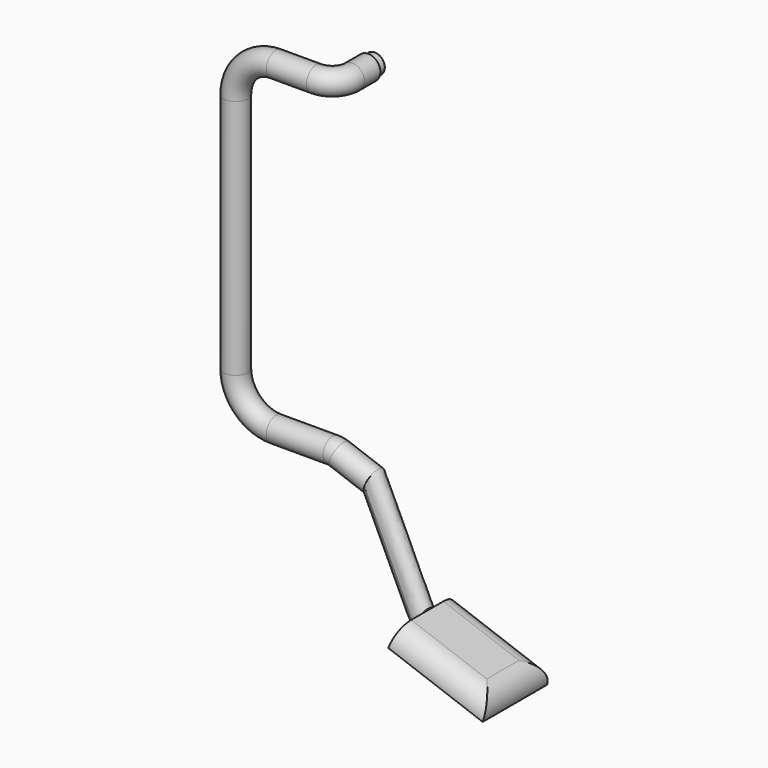
from build123d import *

# Parameters (mm, degrees)
F0_R      = 2.5
F1_DEPTH  = 2
F2_R      = 3
F5_R      = 3
F10_DEPTH = 1
F13_W     = 20
F13_H     = 5
F14_DEPTH = 25
F15_R     = 4.99999


# Not quite as in the source:
# - a fillet or chamfer is up to 0.001 mm smaller than in the source, because OpenCascade refuses the exact size


with BuildPart() as f1:
    # F0 (on Front) → F1 (new body)
    with BuildSketch(Plane.XZ):
        Circle(F0_R)
    extrude(amount=F1_DEPTH)

    # F4: sweep along a path in F3
    with BuildLine(Plane.XY) as f4_path:
        Line((0, -2), (0, -7))
        ThreePointArc((0, -7), (-1.4644660941, -10.5355339059), (-5, -12))
        Line((-5, -12), (-10, -12))
    # F2 (on face) → F4 (sweep)
    with BuildSketch(Plane.XZ.offset(2)):
        Circle(F2_R)
    sweep(path=f4_path.line)

    # F8: sweep along a path in F7
    with BuildLine(Plane.XZ.offset(12)) as f8_path:
        Line((-10, 0), (-15, 0))
        ThreePointArc((-15, 0), (-22.0710678119, -2.9289321881), (-25, -10))
        Line((-25, -10), (-25, -70))
        ThreePointArc((-25, -70), (-22.0710678119, -77.0710678119), (-15, -80))
        Line((-15, -80), (-0.8816349035, -80))
        ThreePointArc((-0.8816349035, -80), (-0.0133940152, -80.0759612349), (0.8284658131, -80.3015368961))
        Line((0.8284658131, -80.3015368961), (9.3969262079, -83.4202014333))
    # F5 (on face) → F8 (sweep)
    with BuildSketch(Plane(origin=(-10, 0, 0), x_dir=(0, -1, 0), z_dir=(-1, 0, 0))):
        with Locations((12, 0)):
            Circle(F5_R)
    sweep(path=f8_path.line)

    # F9 (on face) → F10 (join)
    with BuildSketch(Plane(origin=(35.1084305953, 0, -12.7784237085), x_dir=(0, 1, 0), z_dir=(0.9396926208, 0, -0.3420201433))):
        with BuildLine():
            Line((-9, -75.1754096629), (-15, -75.1754096629))
            ThreePointArc((-15, -75.1754096629), (-12, -78.1754096629), (-9, -75.1754096629))
        make_face()
    extrude(amount=F10_DEPTH)

    # F12: sweep along a path in F11
    with BuildLine(Plane(origin=(-25.7115043875, 0, -70.6417777248), x_dir=(0.9396926208, 0, -0.3420201433), z_dir=(0.3420201433, 0, 0.9396926208))) as f12_path:
        Line((37.3616114661, -12), (70.1276932376, -34.943057454))
    # F9 (on face) + F8_face (on face) → F12 (sweep)
    with BuildSketch(Plane(origin=(35.1084305953, 0, -12.7784237085), x_dir=(0, 1, 0), z_dir=(0.9396926208, 0, -0.3420201433))):
        with BuildLine():
            Line((-9, -75.1754096629), (-15, -75.1754096629))
            ThreePointArc((-15, -75.1754096629), (-12, -78.1754096629), (-9, -75.1754096629))
        make_face()
    with BuildSketch(Plane(origin=(9.3969262079, -12, -83.4202014333), x_dir=(0, 1, 0), z_dir=(0.9396926208, 0, -0.3420201433))):
        with BuildLine():
            ThreePointArc((3, 0), (0, 3), (-3, 0))
            Line((-3, 0), (3, 0))
        make_face()
    sweep(path=f12_path.line)

    # F13 (on face) → F14 (join)
    with BuildSketch(Plane(origin=(65.8984758481, 0, -23.9850836922), x_dir=(0, 1, 0), z_dir=(0.9396926208, 0, -0.3420201433))):
        with Locations((-34.943057454, -75.1754096629)):
            Rectangle(F13_W, F13_H)
    extrude(amount=F14_DEPTH)

    # F15 (radius 5 in the source; OpenCascade refuses exactly that, so slightly less here)
    f15_edges = [f1.edges().sort_by_distance(p)[0] for p in [
        (52.78818, -44.943057, -96.552882),
        (64.534337, -34.943057, -100.828133),
        (52.78818, -24.943057, -96.552882),
    ]]
    fillet(f15_edges, radius=F15_R)


solid = f1.part
